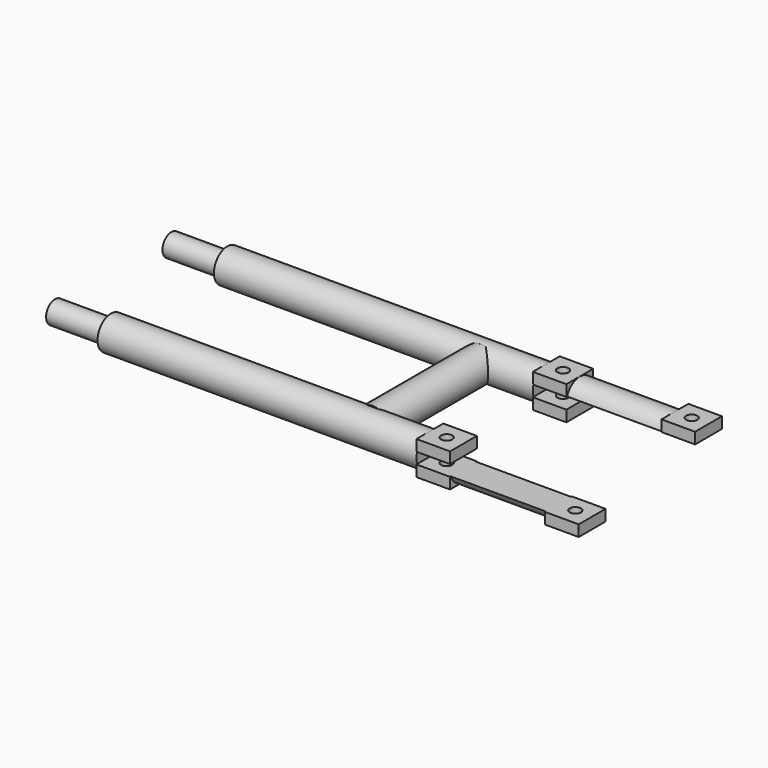
from build123d import *

# Parameters (mm, degrees)
F1_DEPTH      = 15
F2_R          = 7.5
F3_DEPTH      = 240
F4_R          = 7.5
F5_DEPTH      = 30
F5_DEPTH_BACK = 30
F6_W          = 15
F6_H          = 15
F7_DEPTH      = 15
F9_DEPTH      = 40.1
F11_DEPTH     = 54.1
F12_R         = 2.5
F13_DEPTH     = 25
F15_R         = 2.5
F16_DEPTH     = 25
F18_DEPTH     = 25
F17_R         = 7.5
F17_R_2       = 5
F19_DEPTH     = 25


# Not quite as in the source:
# - a feature names something its author has since deleted; it is built from what else it names


with BuildPart() as f1:
    # F0 (on Top) → F1 (new body)
    with BuildSketch(Plane.XY):
        Polygon((-240, -25), (-240, -40), (0, -40), (0, -25), (-100, -25), (-100, 25), (0, 25), (0, 40), (-240, 40), (-240, 25), (-115, 25), (-115, -25), align=None)
    extrude(amount=F1_DEPTH)

    # F2 (on Right) → F3 (intersect)
    with BuildSketch(Plane.YZ):
        with Locations((-32.5, 7.5)):
            Circle(F2_R)
        with Locations((32.5, 7.5)):
            Circle(F2_R)
    extrude(amount=-F3_DEPTH, mode=Mode.INTERSECT)

    # F4 (on Front) → F5 (join, two sides)
    with BuildSketch(Plane.XZ) as f5_sk:
        with Locations((-100, 7.5)):
            Circle(F4_R)
    extrude(amount=F5_DEPTH)
    extrude(f5_sk.sketch, amount=-F5_DEPTH_BACK)

    # F6 (on Top) → F7 (join)
    with BuildSketch(Plane.XY):
        with Locations((-65, 32.5)):
            Rectangle(F6_W, F6_H)
        with Locations((-65, -32.5)):
            Rectangle(F6_W, F6_H)
        with Locations((-7.5, 32.5)):
            Rectangle(F6_W, F6_H)
        with Locations((-7.5, -32.5)):
            Rectangle(F6_W, F6_H)
    extrude(amount=F7_DEPTH)

    # F8 (on Front) → F9 (cut)
    with BuildSketch(Plane.XZ):
        Polygon((0, 0), (0, 10), (-72.5, 10), (-72.5, 5), (-57.5, 5), (-57.5, 0), align=None)
    extrude(amount=-F9_DEPTH, mode=Mode.SUBTRACT)

    # F10 (on Front) → F11 (cut)
    with BuildSketch(Plane.XZ):
        Polygon((0, 5), (0, 15), (-57.5, 15), (-57.5, 10), (-72.5, 10), (-72.5, 5), (-57.5, 5), align=None)
    extrude(amount=F11_DEPTH, mode=Mode.SUBTRACT)

    # F12 (on Top) → F13 (cut)
    with BuildSketch(Plane.XY):
        with Locations((-65, 32.5)):
            Circle(F12_R)
        with Locations((-65, -32.5)):
            Circle(F12_R)
        with Locations((-7.5, -32.5)):
            Circle(F12_R)
        with Locations((-7.5, 32.5)):
            Circle(F12_R)
    extrude(amount=F13_DEPTH, mode=Mode.SUBTRACT)

    # F15 (on offset) → F16 (cut)
    with BuildSketch(Plane(origin=(-240, 0, 0), x_dir=(0, -1, 0), z_dir=(-1, 0, 0))):
        with Locations((-32.5, 7.5)):
            Circle(F15_R)
        with Locations((32.5, 7.5)):
            Circle(F15_R)
    extrude(amount=-F16_DEPTH, mode=Mode.SUBTRACT)

    # F0 (on Top) → F18 (cut)
    with BuildSketch(Plane.XY):
        Polygon((-240, -25), (-240, -40), (0, -40), (0, -25), (-100, -25), (-100, 25), (0, 25), (0, 40), (-240, 40), (-240, 25), (-115, 25), (-115, -25), align=None)
    extrude(amount=-F18_DEPTH, mode=Mode.SUBTRACT)

    # F17 (on offset) → F19 (cut)
    with BuildSketch(Plane(origin=(-240, 0, 0), x_dir=(0, -1, 0), z_dir=(-1, 0, 0))):
        with Locations((-32.5, 7.5)):
            Circle(F17_R)
        with Locations((-32.5, 7.5)):
            Circle(F17_R_2, mode=Mode.SUBTRACT)
        with Locations((32.5, 7.5)):
            Circle(F17_R)
        with Locations((32.5, 7.5)):
            Circle(F17_R_2, mode=Mode.SUBTRACT)
    extrude(amount=-F19_DEPTH, mode=Mode.SUBTRACT)


solid = f1.part
